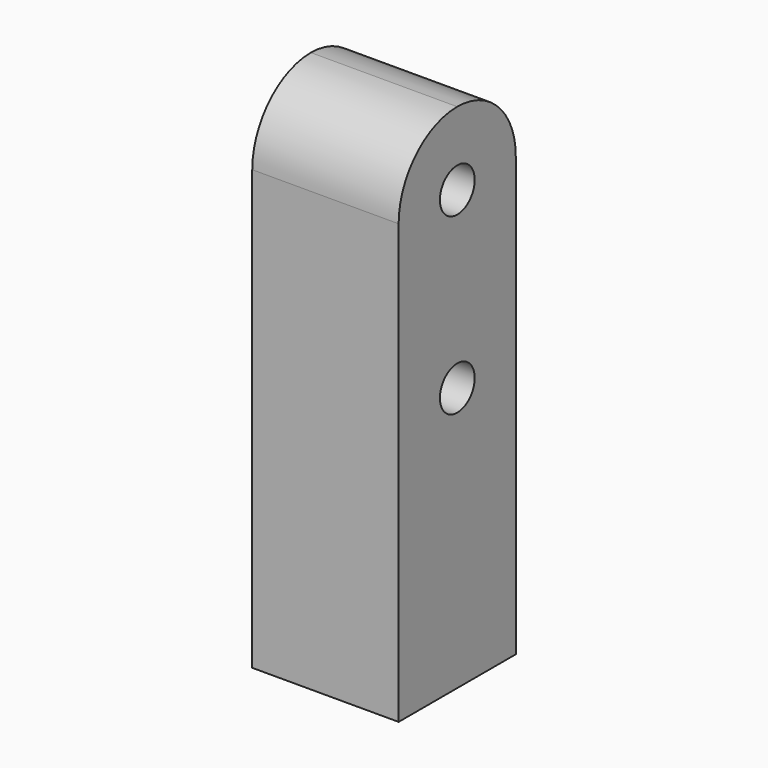
from build123d import *

# Parameters (mm, degrees)
F0_W          = 13.3
F0_H          = 13.3
F0_W_2        = 10.3
F0_H_2        = 10.3
F1_DEPTH      = 20
F2_DEPTH      = 1.5
F3_W          = 4
F3_H          = 13.3
F3_W_2        = 5.3
F4_DEPTH      = 25
F5_T1_DEPTH   = 46.6
F6_R          = 1.975
F7_DEPTH      = 25
F7_DEPTH_BACK = 25


# Not quite as in the source:
# - a fillet or chamfer that OpenCascade refuses, or shapes differently, is made with other operations: its cross-section is extruded or revolved along the edge and cut away or added


with BuildPart() as f1:
    # F0 (on Top) → F1 (new body)
    with BuildSketch(Plane.XY):
        Rectangle(F0_W, F0_H)
        Rectangle(F0_W_2, F0_H_2, mode=Mode.SUBTRACT)
    extrude(amount=-F1_DEPTH)

    # F0 (on Top) → F2 (join)
    with BuildSketch(Plane.XY):
        Rectangle(F0_W, F0_H)
        Rectangle(F0_W_2, F0_H_2, mode=Mode.SUBTRACT)
        Rectangle(F0_W_2, F0_H_2)
    extrude(amount=F2_DEPTH)

    # F3 (on face) → F4 (join)
    with BuildSketch(Plane.XY.offset(1.5)):
        with Locations((-4.65, 0)):
            Rectangle(F3_W, F3_H)
        with Locations((4.65, 0)):
            Rectangle(F3_W, F3_H)
        Rectangle(F3_W_2, F3_H)
    extrude(amount=F4_DEPTH)

    # F5: fillet of radius 6.66 on 2 edges, made by hand

    # F5_s2 → F5_t1 (cut)
    with BuildSketch(Plane.YZ.offset(-23.3)):
        with BuildLine():
            ThreePointArc((-0.01, 26.5), (4.6993311627, 24.5493311627), (6.65, 19.84))
            Line((6.65, 19.84), (6.65, 26.5))
            Line((6.65, 26.5), (-0.01, 26.5))
        make_face()
        with BuildLine():
            ThreePointArc((-6.65, 19.84), (-4.6993311627, 24.5493311627), (0.01, 26.5))
            Line((0.01, 26.5), (-6.65, 26.5))
            Line((-6.65, 26.5), (-6.65, 19.84))
        make_face()
    extrude(amount=F5_T1_DEPTH, mode=Mode.SUBTRACT)

    # F6 (on face) → F7 (cut, two sides)
    with BuildSketch(Plane.YZ.offset(6.65)) as f7_sk:
        with Locations((0.01, 4)):
            Circle(F6_R)
        with Locations((0.01, 19.84)):
            Circle(F6_R)
    extrude(amount=-F7_DEPTH, mode=Mode.SUBTRACT)
    extrude(f7_sk.sketch, amount=F7_DEPTH_BACK, mode=Mode.SUBTRACT)


solid = f1.part
